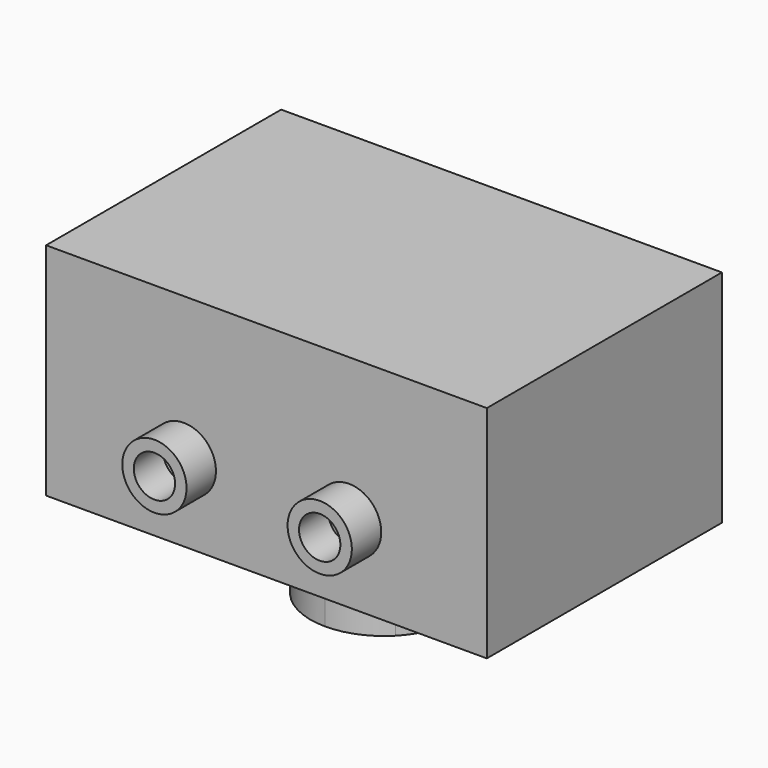
from build123d import *

# Parameters (mm, degrees)
F1_DEPTH = 152.4
F2_DEPTH = 50.8
F4_DEPTH = 25.4
F5_W     = 100.7168591022
F5_H     = 42.3558056355
F6_DEPTH = 6.35
F7_SIZE  = 2.54


with BuildPart() as f1:
    # F0 (on Top) → F1 (new body)
    with BuildSketch(Plane.XY):
        with BuildLine():
            Line((152.4, 0), (50.8, 0))
            ThreePointArc((50.8, 0), (47.0438920676, -19.1706082098), (36.3310149947, -35.5063001375))
            ThreePointArc((36.3310149947, -35.5063001375), (19.7093880297, -46.820722159), (0, -50.8))
            Line((0, -50.8), (0, -101.6))
            Line((0, -101.6), (152.4, -101.6))
            Line((152.4, -101.6), (152.4, 0))
        make_face()
        with BuildLine():
            ThreePointArc((0, 50.8), (35.9210244843, 35.9210244843), (50.8, 0))
            Line((50.8, 0), (152.4, 0))
            Line((152.4, 0), (152.4, 101.6))
            Line((152.4, 101.6), (0, 101.6))
            Line((0, 101.6), (0, 50.8))
        make_face()
        with BuildLine():
            ThreePointArc((0, -50.8), (-50.8, 0), (0, 50.8))
            Line((0, 50.8), (0, 101.6))
            Line((0, 101.6), (-152.4, 101.6))
            Line((-152.4, 101.6), (-152.4, -101.6))
            Line((-152.4, -101.6), (0, -101.6))
            Line((0, -101.6), (0, -50.8))
        make_face()
        with BuildLine():
            Line((0, -50.8), (0, 0))
            Line((0, 0), (0, 50.8))
            ThreePointArc((0, 50.8), (-50.8, 0), (0, -50.8))
        make_face()
        with BuildLine():
            Line((0, 50.8), (0, 0))
            Line((0, 0), (50.8, 0))
            ThreePointArc((50.8, 0), (35.9210244843, 35.9210244843), (0, 50.8))
        make_face()
        with BuildLine():
            Line((36.3310149947, -35.5063001375), (0, 0))
            Line((0, 0), (0, -50.8))
            ThreePointArc((0, -50.8), (19.7093880297, -46.820722159), (36.3310149947, -35.5063001375))
        make_face()
        with BuildLine():
            Line((50.8, 0), (0, 0))
            Line((0, 0), (36.3310149947, -35.5063001375))
            ThreePointArc((36.3310149947, -35.5063001375), (47.0438920676, -19.1706082098), (50.8, 0))
        make_face()
    extrude(amount=F1_DEPTH)

    # F0 (on Top) → F2 (join)
    with BuildSketch(Plane.XY):
        with BuildLine():
            Line((36.3310149947, -35.5063001375), (0, 0))
            Line((0, 0), (0, -50.8))
            ThreePointArc((0, -50.8), (19.7093880297, -46.820722159), (36.3310149947, -35.5063001375))
        make_face()
        with BuildLine():
            Line((50.8, 0), (0, 0))
            Line((0, 0), (36.3310149947, -35.5063001375))
            ThreePointArc((36.3310149947, -35.5063001375), (47.0438920676, -19.1706082098), (50.8, 0))
        make_face()
        with BuildLine():
            Line((0, 50.8), (0, 0))
            Line((0, 0), (50.8, 0))
            ThreePointArc((50.8, 0), (35.9210244843, 35.9210244843), (0, 50.8))
        make_face()
        with BuildLine():
            Line((0, -50.8), (0, 0))
            Line((0, 0), (0, 50.8))
            ThreePointArc((0, 50.8), (-50.8, 0), (0, -50.8))
        make_face()
    extrude(amount=-F2_DEPTH)

    # F3 (on face) → F4 (join)
    with BuildSketch(Plane.XZ.offset(101.6)):
        with BuildLine():
            ThreePointArc((34.925, 53.1082823873), (57.15, 30.8832823873), (79.375, 53.1082823873))
            Line((79.375, 53.1082823873), (71.4375, 53.1082823873))
            ThreePointArc((71.4375, 53.1082823873), (57.15, 38.8207823873), (42.8625, 53.1082823873))
            Line((42.8625, 53.1082823873), (34.925, 53.1082823873))
        make_face()
        with BuildLine():
            Line((71.4375, 53.1082823873), (79.375, 53.1082823873))
            ThreePointArc((79.375, 53.1082823873), (57.15, 75.3332823873), (34.925, 53.1082823873))
            Line((34.925, 53.1082823873), (42.8625, 53.1082823873))
            ThreePointArc((42.8625, 53.1082823873), (57.15, 67.3957823873), (71.4375, 53.1082823873))
        make_face()
        with BuildLine():
            ThreePointArc((-34.925, 53.1082823873), (-57.15, 75.3332823873), (-79.375, 53.1082823873))
            Line((-79.375, 53.1082823873), (-71.4375, 53.1082823873))
            ThreePointArc((-71.4375, 53.1082823873), (-57.15, 67.3957823873), (-42.8625, 53.1082823873))
            Line((-42.8625, 53.1082823873), (-34.925, 53.1082823873))
        make_face()
        with BuildLine():
            Line((-71.4375, 53.1082823873), (-79.375, 53.1082823873))
            ThreePointArc((-79.375, 53.1082823873), (-57.15, 30.8832823873), (-34.925, 53.1082823873))
            Line((-34.925, 53.1082823873), (-42.8625, 53.1082823873))
            ThreePointArc((-42.8625, 53.1082823873), (-57.15, 38.8207823873), (-71.4375, 53.1082823873))
        make_face()
    extrude(amount=F4_DEPTH)


with BuildPart() as f6:
    # F5 (on face) → F6 (new body)
    with BuildSketch(Plane(origin=(0, 101.6, 0), x_dir=(-1, 0, 0), z_dir=(0, 1, 0))):
        with Locations((66.9497698545, 98.8216623664)):
            Rectangle(F5_W, F5_H)
    extrude(amount=F6_DEPTH)

    # F7
    f7_edges = [f6.edges().sort_by_distance(p)[0] for p in [
        (-66.94977, 107.95, 119.999565),
        (-117.308199, 107.95, 98.821662),
        (-16.59134, 107.95, 98.821662),
        (-66.94977, 107.95, 77.64376),
    ]]
    chamfer(f7_edges, length=F7_SIZE)


solid = Compound([f1.part, f6.part])
